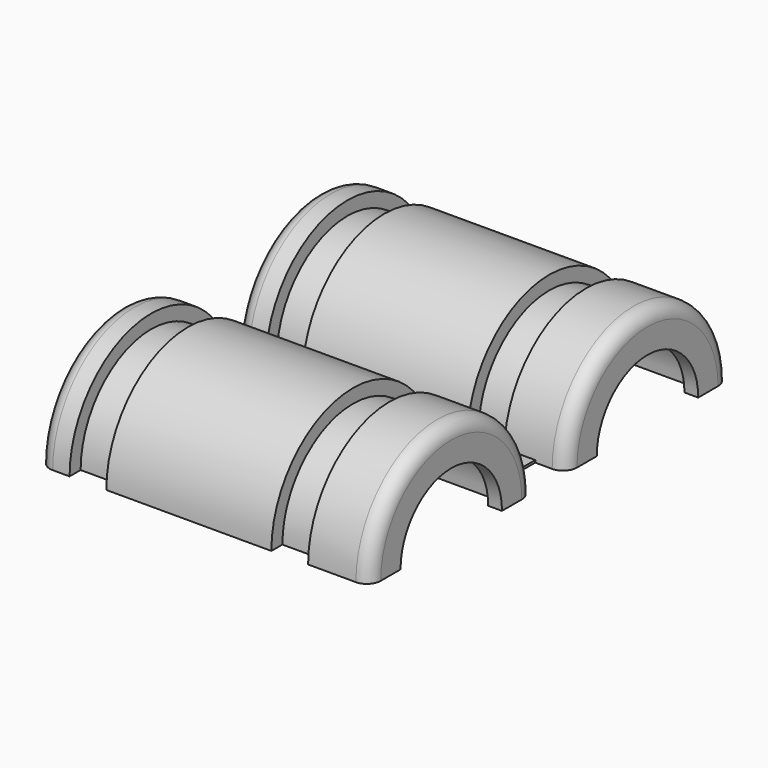
from build123d import *

# Parameters (mm, degrees)
F2_ANGLE = 180
F3_ANGLE = 180
F1_W     = 1.8325150013
F1_H     = 5.3774006665
F1_W_2   = 1.83251407
F1_H_2   = 5.3300224245
F4_DEPTH = 0.25


# Not quite as in the source:
# - ends of sketch curves that miss each other by under 0.0002 mm in the source are joined
# - a feature names something its author has since deleted; it is built from what else it names


with BuildPart() as f2:
    # F0 (on Top) → F2 (revolve)
    with BuildSketch(Plane.XY):
        with BuildLine():
            Line((34.5, 8.2), (34.5, 9.6))
            ThreePointArc((34.5, 9.6), (34.0606601718, 10.6606601718), (33, 11.1))
            Line((33, 11.1), (27.8003929108, 11.1000006409))
            Line((27.8003929108, 11.1000006409), (27.8003929108, 9.600000456))
            Line((27.8003929108, 9.600000456), (23.8003929108, 9.600000456))
            Line((23.8003929108, 9.600000456), (23.8003929108, 11.100000456))
            Line((23.8003929108, 11.100000456), (5.8400444046, 11.0999997705))
            Line((5.8400444046, 11.0999997705), (5.8400444046, 9.6))
            Line((5.8400444046, 9.6), (1.8400444046, 9.6))
            Line((1.8400444046, 9.6), (1.8400444046, 11.1))
            Line((1.8400444046, 11.1), (0, 11.1))
            ThreePointArc((0, 11.1), (-1.0606601718, 10.6606601718), (-1.5, 9.6))
            Line((-1.5, 9.6), (-1.5, 6.9))
            Line((-1.5, 6.9), (0, 6.9))
            Line((0, 6.9), (0, 8.8))
            Line((0, 8.8), (12.2141037136, 8.2))
            Line((12.2141037136, 8.2), (33, 8.2))
            Line((33, 8.2), (33, 6.9))
            Line((33, 6.9), (34.5, 6.9))
            Line((34.5, 6.9), (34.5, 8.2))
        make_face()
    revolve(axis=Axis((17.25, 0, 0), (1, 0, 0)), revolution_arc=F2_ANGLE)



with BuildPart() as f3:
    # F0 (on Top) → F3 (revolve)
    with BuildSketch(Plane.XY):
        with BuildLine():
            Line((34.5, 17.1004687339), (34.5, 18.5004687339))
            Line((34.5, 18.5004687339), (34.5, 19.8004687339))
            Line((34.5, 19.8004687339), (33, 19.8004687339))
            Line((33, 19.8004687339), (33, 18.5004687339))
            Line((33, 18.5004687339), (12.2141037136, 18.5004687339))
            Line((12.2141037136, 18.5004687339), (0, 17.9004687339))
            Line((0, 17.9004687339), (0, 19.8004687339))
            Line((0, 19.8004687339), (-1.5, 19.8004687339))
            Line((-1.5, 19.8004687339), (-1.5, 17.1004687339))
            ThreePointArc((-1.5, 17.1004687339), (-1.0606601718, 16.0398085621), (0, 15.6004687339))
            Line((0, 15.6004687339), (1.8400444046, 15.6004687339))
            Line((1.8400444046, 15.6004687339), (1.8400444046, 17.1004687339))
            Line((1.8400444046, 17.1004687339), (5.8400444046, 17.1004687339))
            Line((5.8400444046, 17.1004687339), (5.8400444046, 15.6004687339))
            Line((5.8400444046, 15.6004687339), (23.8003929108, 15.6004682779))
            Line((23.8003929108, 15.6004682779), (23.8003929108, 17.1004682779))
            Line((23.8003929108, 17.1004682779), (27.8003929108, 17.1004682779))
            Line((27.8003929108, 17.1004682779), (27.8003929108, 15.6004680931))
            Line((27.8003929108, 15.6004680931), (33, 15.6004687339))
            ThreePointArc((33, 15.6004687339), (34.0606601718, 16.0398085621), (34.5, 17.1004687339))
        make_face()
    revolve(axis=Axis((17.25, 26.7004687339, 0), (-1, 0, 0)), revolution_arc=F3_ANGLE)


with BuildPart() as f2_1:
    add(f2.part)

    add(f3.part)  # F4 merges F3
    # F1 (on Top) → F4 (join)
    with BuildSketch(Plane.XY):
        with Locations((30.2449278533, 13.3801726624)):
            Rectangle(F1_W, F1_H)
        with Locations((8.218171075, 13.3564835414)):
            Rectangle(F1_W_2, F1_H_2)
    extrude(amount=F4_DEPTH)


solid = f2_1.part
